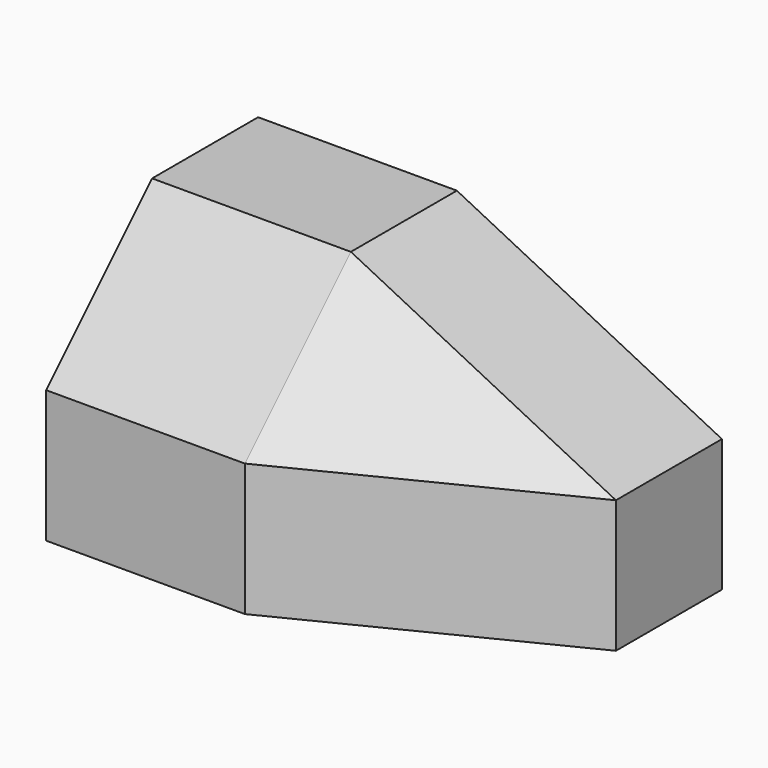
from build123d import *

# Parameters (mm, degrees)
F0_W     = 70
F0_H     = 40
F1_DEPTH = 40
F2_SIZE  = 20
F3_SIZE2 = 20
F3_SIZE  = 40
F4_SIZE2 = 20
F4_SIZE  = 40
F7_DEPTH = 26.6676666667


with BuildPart() as f1:
    # F0 (on Top) → F1 (new body)
    with BuildSketch(Plane.XY):
        with Locations((35, 20)):
            Rectangle(F0_W, F0_H)
    extrude(amount=F1_DEPTH)

    # F2
    f2_edges = [f1.edges().sort_by_distance(p)[0] for p in [
        (35, 0, 40),
    ]]
    chamfer(f2_edges, length=F2_SIZE)

    # F3
    f3_edges = [f1.edges().sort_by_distance(p)[0] for p in [
        (70, 30, 40),
    ]]
    f3_side = f1.faces().sort_by_distance((35, 30, 40))[0]
    chamfer(f3_edges, length=F3_SIZE, length2=F3_SIZE2, reference=f3_side)

    # F4
    f4_edges = [f1.edges().sort_by_distance(p)[0] for p in [
        (70, 0, 10),
    ]]
    f4_side = f1.faces().sort_by_distance((35, 0, 10))[0]
    chamfer(f4_edges, length=F4_SIZE, length2=F4_SIZE2, reference=f4_side)

    # F6 (on face) → F7 (cut, through all)
    with BuildSketch(Plane(origin=(7.7777777778, -15.5555555556, 15.5555555556), x_dir=(0.9428090416, 0.2357022604, -0.2357022604), z_dir=(-0.3333333333, 0.6666666667, -0.6666666667))):
        Polygon((23.5702260396, -14.1421356237), (23.5702260396, -42.4264068712), (65.9966329107, -28.2842712475), align=None)
    extrude(amount=-F7_DEPTH, mode=Mode.SUBTRACT)


solid = f1.part
